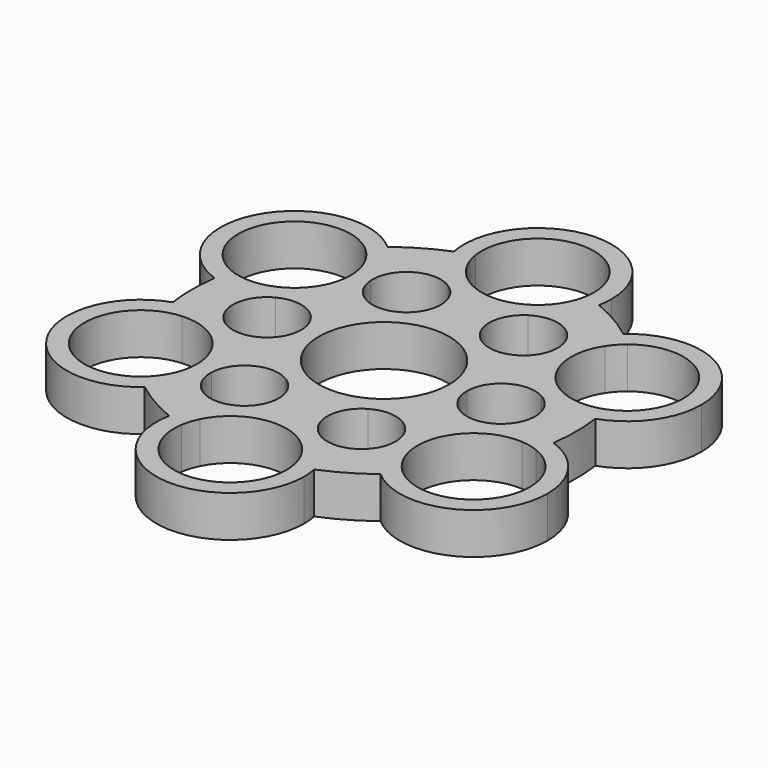
from build123d import *

# Parameters (mm, degrees)
F0_R     = 11
F1_DEPTH = 7


with BuildPart() as f1:
    # F0 (on Top) → F1 (new body)
    with BuildSketch(Plane.XY):
        with BuildLine():
            ThreePointArc((7.0000001006, -12.1243555949), (12.124355682, -6.9999999497), (14, 0))
            ThreePointArc((14, 0), (12.1243557011, 6.9999999166), (7.0000001668, 12.1243555567))
            ThreePointArc((7.0000001668, 12.1243555567), (0.1361246737, 13.9993382013), (-6.7629128968, 12.2581813149))
            ThreePointArc((-6.7629128968, 12.2581813149), (-6.99546954, 12.1165086661), (-7.2344399745, 11.9859450297))
            ThreePointArc((-7.2344399745, 11.9859450297), (-12.191844808, 6.881781759), (-14, 0))
            ThreePointArc((-14, 0), (-12.1243555958, -7.000000099), (-6.999999802, -12.1243557673))
            ThreePointArc((-6.999999802, -12.1243557673), (1.724e-07, -14), (7.0000001006, -12.1243555949))
        make_face()
        Circle(F0_R, mode=Mode.SUBTRACT)
        with BuildLine():
            ThreePointArc((22.4231761247, -5.1368869024), (16.769566617, -4.9329885231), (14, 0))
            ThreePointArc((14, 0), (12.124355682, -6.9999999497), (7.0000001006, -12.1243555949))
            ThreePointArc((7.0000001006, -12.1243555949), (12.6568763598, -12.0563762611), (15.6602625749, -16.8505958477))
            ThreePointArc((15.6602625749, -16.8505958477), (17.3205082906, -9.9999996277), (22.4231761247, -5.1368869024))
        make_face()
        with BuildLine():
            ThreePointArc((7.0000001668, 12.1243555567), (12.1243557011, 6.9999999166), (14, 0))
            ThreePointArc((14, 0), (16.769566627, 4.9329885292), (22.4231761455, 5.1368868917))
            ThreePointArc((22.4231761455, 5.1368868917), (17.3205082443, 9.9999997079), (15.6602625849, 16.8505960559))
            ThreePointArc((15.6602625849, 16.8505960559), (12.6568764848, 12.0563763294), (7.0000001668, 12.1243555567))
        make_face()
        with BuildLine():
            ThreePointArc((-6.7629128968, 12.2581813149), (0.1361246737, 13.9993382013), (7.0000001668, 12.1243555567))
            ThreePointArc((7.0000001668, 12.1243555567), (4.1126899405, 16.9893645646), (6.7629130014, 21.9874832825))
            ThreePointArc((6.7629130014, 21.9874832825), (0.0018890383, 20.0000001427), (-6.759735325, 21.9854396984))
            ThreePointArc((-6.759735325, 21.9854396984), (-4.8119543875, 19.8928592028), (-4.1050678819, 17.1228311923))
            ThreePointArc((-4.1050678819, 17.1228311923), (-4.8128595342, 14.3511458497), (-6.7629128968, 12.2581813149))
        make_face()
        with BuildLine():
            ThreePointArc((6.7629128862, -21.9874832084), (4.1126899412, -16.9893645344), (7.0000001006, -12.1243555949))
            ThreePointArc((7.0000001006, -12.1243555949), (1.724e-07, -14), (-6.999999802, -12.1243557673))
            ThreePointArc((-6.999999802, -12.1243557673), (-4.8851208082, -14.2392348866), (-4.1110213762, -17.1282134114))
            ThreePointArc((-4.1110213762, -17.1282134114), (-4.8171414782, -19.8961111559), (-6.7629128995, -21.987483217))
            ThreePointArc((-6.7629128995, -21.987483217), (-7.9e-09, -20), (6.7629128862, -21.9874832084))
        make_face()
        with BuildLine():
            ThreePointArc((15.6602625849, 16.8505960559), (17.3205082443, 9.9999997079), (22.4231761455, 5.1368868917))
            ThreePointArc((22.4231761455, 5.1368868917), (25.7437624558, 3.9829672479), (29.2543281187, 3.7992481264))
            ThreePointArc((29.2543281187, 3.7992481264), (29.0218126442, 5.2900274902), (28.7133790239, 6.7669686736))
            ThreePointArc((28.7133790239, 6.7669686736), (19.918584287, 11.5), (20.2170562899, 21.4830313264))
            ThreePointArc((20.2170562899, 21.4830313264), (19.0922045153, 22.4886132686), (17.9174094521, 23.4353672582))
            ThreePointArc((17.9174094521, 23.4353672582), (16.3212319377, 20.3032683327), (15.6602625849, 16.8505960559))
        make_face()
        with BuildLine():
            ThreePointArc((29.2543281187, 3.7992481264), (25.7437624558, 3.9829672479), (22.4231761455, 5.1368868917))
            ThreePointArc((22.4231761455, 5.1368868917), (24.7109457768, 3.0083906207), (25.5559144953, 0))
            ThreePointArc((25.5559144953, 0), (24.7109457708, -3.0083906307), (22.4231761247, -5.1368869024))
            ThreePointArc((22.4231761247, -5.1368869024), (25.7437624444, -3.9829672502), (29.2543281187, -3.7992481264))
            ThreePointArc((29.2543281187, -3.7992481264), (29.5, 0), (29.2543281187, 3.7992481264))
        make_face()
        with BuildLine():
            ThreePointArc((29.2543281187, -3.7992481264), (25.7437624444, -3.9829672502), (22.4231761247, -5.1368869024))
            ThreePointArc((22.4231761247, -5.1368869024), (17.3205082906, -9.9999996277), (15.6602625749, -16.8505958477))
            ThreePointArc((15.6602625749, -16.8505958477), (16.3212319039, -20.3032682341), (17.9174094521, -23.4353672582))
            ThreePointArc((17.9174094521, -23.4353672582), (19.0922045153, -22.4886132686), (20.2170562899, -21.4830313264))
            ThreePointArc((20.2170562899, -21.4830313264), (19.918584287, -11.5), (28.7133790239, -6.7669686736))
            ThreePointArc((28.7133790239, -6.7669686736), (29.0218126442, -5.2900274902), (29.2543281187, -3.7992481264))
        make_face()
        with BuildLine():
            ThreePointArc((-6.759735325, 21.9854396984), (0.0018890383, 20.0000001427), (6.7629130014, 21.9874832825))
            ThreePointArc((6.7629130014, 21.9874832825), (9.422530203, 24.2862356636), (11.3369186666, 27.2346153846))
            ThreePointArc((11.3369186666, 27.2346153846), (9.9296081288, 27.7786407588), (8.496322734, 28.25))
            ThreePointArc((8.496322734, 28.25), (0, 23), (-8.496322734, 28.25))
            ThreePointArc((-8.496322734, 28.25), (-9.9296081288, 27.7786407588), (-11.3369186666, 27.2346153846))
            ThreePointArc((-11.3369186666, 27.2346153846), (-9.4212888061, 24.2848117957), (-6.759735325, 21.9854396984))
        make_face()
        with BuildLine():
            ThreePointArc((11.3369186666, 27.2346153846), (9.422530203, 24.2862356636), (6.7629130014, 21.9874832825))
            ThreePointArc((6.7629130014, 21.9874832825), (12.6568764214, 22.2000505281), (15.6669358715, 17.1282134114))
            ThreePointArc((15.6669358715, 17.1282134114), (15.6652673089, 16.9893646368), (15.6602625849, 16.8505960559))
            ThreePointArc((15.6602625849, 16.8505960559), (16.3212319377, 20.3032683327), (17.9174094521, 23.4353672582))
            ThreePointArc((17.9174094521, 23.4353672582), (14.75, 25.5477494116), (11.3369186666, 27.2346153846))
        make_face()
        with BuildLine():
            ThreePointArc((-15.6602625894, -16.850596149), (-12.6568763408, -12.0563762508), (-6.999999802, -12.1243557673))
            ThreePointArc((-6.999999802, -12.1243557673), (-12.1243555958, -7.000000099), (-14, 0))
            ThreePointArc((-14, 0), (-16.7695666992, -4.9329885732), (-22.4231762959, -5.1368868142))
            ThreePointArc((-22.4231762959, -5.1368868143), (-17.4738268273, -9.741663676), (-15.645825623, -16.25))
            ThreePointArc((-15.645825623, -16.25), (-15.6494353858, -16.5503848199), (-15.6602625894, -16.850596149))
        make_face()
        with BuildLine():
            ThreePointArc((17.9174094521, -23.4353672582), (16.3212319039, -20.3032682341), (15.6602625749, -16.8505958477))
            ThreePointArc((15.6602625749, -16.8505958477), (15.6652673064, -16.9893645326), (15.6669358715, -17.1282134114))
            ThreePointArc((15.6669358715, -17.1282134114), (12.6568763613, -22.2000505609), (6.7629128862, -21.9874832084))
            ThreePointArc((6.7629128862, -21.9874832084), (9.422530158, -24.286235612), (11.3369186666, -27.2346153846))
            ThreePointArc((11.3369186666, -27.2346153846), (14.75, -25.5477494116), (17.9174094521, -23.4353672582))
        make_face()
        with BuildLine():
            ThreePointArc((11.3369186666, -27.2346153846), (9.422530158, -24.286235612), (6.7629128862, -21.9874832084))
            ThreePointArc((6.7629128862, -21.9874832084), (-7.9e-09, -20), (-6.7629128995, -21.987483217))
            ThreePointArc((-6.7629128995, -21.987483217), (-9.4225301632, -24.286235618), (-11.3369186666, -27.2346153846))
            ThreePointArc((-11.3369186666, -27.2346153846), (-9.9296081288, -27.7786407588), (-8.496322734, -28.25))
            ThreePointArc((-8.496322734, -28.25), (0, -23), (8.496322734, -28.25))
            ThreePointArc((8.496322734, -28.25), (9.9296081288, -27.7786407588), (11.3369186666, -27.2346153846))
        make_face()
        with BuildLine():
            ThreePointArc((28.7133790239, 6.7669686736), (29.0218126442, 5.2900274902), (29.2543281187, 3.7992481264))
            ThreePointArc((29.2543281187, 3.7992481264), (30.7447425948, 4.0231594198), (32.1973755284, 4.4248174067))
            ThreePointArc((32.1973755284, 4.4248174067), (31.9549148923, 5.9273446187), (31.642376555, 7.4168730576))
            ThreePointArc((31.642376555, 7.4168730576), (30.2036958653, 6.9755636254), (28.7133790239, 6.7669686736))
        make_face()
        with BuildLine():
            ThreePointArc((32.1973755284, 4.4248174067), (30.7447425948, 4.0231594198), (29.2543281187, 3.7992481264))
            ThreePointArc((29.2543281187, 3.7992481264), (29.5, 0), (29.2543281187, -3.7992481264))
            ThreePointArc((29.2543281187, -3.7992481264), (30.7447425948, -4.0231594198), (32.1973755284, -4.4248174067))
            ThreePointArc((32.1973755284, -4.4248174067), (32.5, 0), (32.1973755284, 4.4248174067))
        make_face()
        with BuildLine():
            ThreePointArc((32.1973755284, -4.4248174067), (30.7447425948, -4.0231594198), (29.2543281187, -3.7992481264))
            ThreePointArc((29.2543281187, -3.7992481264), (29.0218126442, -5.2900274902), (28.7133790239, -6.7669686736))
            ThreePointArc((28.7133790239, -6.7669686736), (30.2036958653, -6.9755636254), (31.642376555, -7.4168730576))
            ThreePointArc((31.642376555, -7.4168730576), (31.9549148923, -5.9273446187), (32.1973755284, -4.4248174067))
        make_face()
        with BuildLine():
            ThreePointArc((-14, 0), (-12.191844808, 6.881781759), (-7.2344399745, 11.9859450297))
            ThreePointArc((-7.2344399745, 11.9859450297), (-12.7746372788, 12.1155647212), (-15.660081627, 16.8468223075))
            ThreePointArc((-15.660081627, 16.8468223075), (-15.6493901322, 16.5484962731), (-15.645825623, 16.25))
            ThreePointArc((-15.645825623, 16.25), (-17.473826823, 9.7416636832), (-22.423176281, 5.1368868219))
            ThreePointArc((-22.423176281, 5.1368868219), (-16.769566692, 4.9329885689), (-14, 0))
        make_face()
        with BuildLine():
            ThreePointArc((-15.660081627, 16.8468223075), (-12.7762728806, 22.1291537044), (-6.759735325, 21.9854396984))
            ThreePointArc((-6.759735325, 21.9854396984), (-9.4212888061, 24.2848117957), (-11.3369186666, 27.2346153846))
            ThreePointArc((-11.3369186666, 27.2346153846), (-14.75, 25.5477494116), (-17.9174094521, 23.4353672582))
            ThreePointArc((-17.9174094521, 23.4353672582), (-16.3206195291, 20.3014813138), (-15.660081627, 16.8468223075))
        make_face()
        with BuildLine():
            ThreePointArc((8.496322734, 28.25), (9.9296081288, 27.7786407588), (11.3369186666, 27.2346153846))
            ThreePointArc((11.3369186666, 27.2346153846), (11.8882130364, 28.6373078299), (12.2666834829, 30.0961538462))
            ThreePointArc((12.2666834829, 30.0961538462), (10.8442264294, 30.6374403818), (9.3979877929, 31.1115384615))
            ThreePointArc((9.3979877929, 31.1115384615), (9.0608326273, 29.6449497203), (8.496322734, 28.25))
        make_face()
        with BuildLine():
            ThreePointArc((12.2666834829, 30.0961538462), (11.8882130364, 28.6373078299), (11.3369186666, 27.2346153846))
            ThreePointArc((11.3369186666, 27.2346153846), (14.75, 25.5477494116), (17.9174094521, 23.4353672582))
            ThreePointArc((17.9174094521, 23.4353672582), (18.8565295584, 24.61414841), (19.9306920455, 25.6713364394))
            ThreePointArc((19.9306920455, 25.6713364394), (16.25, 28.145825623), (12.2666834829, 30.0961538462))
        make_face()
        with BuildLine():
            ThreePointArc((19.9306920455, 25.6713364394), (18.8565295584, 24.61414841), (17.9174094521, 23.4353672582))
            ThreePointArc((17.9174094521, 23.4353672582), (19.0922045153, 22.4886132686), (20.2170562899, 21.4830313264))
            ThreePointArc((20.2170562899, 21.4830313264), (21.142863238, 22.6693860948), (22.244388762, 23.6946654039))
            ThreePointArc((22.244388762, 23.6946654039), (21.1106884629, 24.7100957631), (19.9306920455, 25.6713364394))
        make_face()
        with BuildLine():
            ThreePointArc((-6.7629128995, -21.987483217), (-12.7779571757, -22.1320712114), (-15.6602625894, -16.850596149))
            ThreePointArc((-15.6602625894, -16.850596149), (-16.3212319528, -20.3032683768), (-17.9174094521, -23.4353672582))
            ThreePointArc((-17.9174094521, -23.4353672582), (-14.75, -25.5477494116), (-11.3369186666, -27.2346153846))
            ThreePointArc((-11.3369186666, -27.2346153846), (-9.4225301632, -24.286235618), (-6.7629128995, -21.987483217))
        make_face()
        with BuildLine():
            ThreePointArc((-17.9174094521, -23.4353672582), (-16.3212319528, -20.3032683768), (-15.6602625894, -16.850596149))
            ThreePointArc((-15.6602625894, -16.850596149), (-15.6494353858, -16.5503848199), (-15.645825623, -16.25))
            ThreePointArc((-15.645825623, -16.25), (-17.4738268273, -9.741663676), (-22.4231762959, -5.1368868143))
            ThreePointArc((-22.4231762959, -5.1368868143), (-25.7437625388, -3.9829672317), (-29.2543281187, -3.7992481264))
            ThreePointArc((-29.2543281187, -3.7992481264), (-29.0218126442, -5.2900274902), (-28.7133790239, -6.7669686736))
            ThreePointArc((-28.7133790239, -6.7669686736), (-21.6320616308, -9.3347358218), (-18.645825623, -16.25))
            ThreePointArc((-18.645825623, -16.25), (-19.0471084424, -18.9819124561), (-20.2170562899, -21.4830313264))
            ThreePointArc((-20.2170562899, -21.4830313264), (-19.0922045153, -22.4886132686), (-17.9174094521, -23.4353672582))
        make_face()
        with BuildLine():
            ThreePointArc((20.2170562899, -21.4830313264), (19.0922045153, -22.4886132686), (17.9174094521, -23.4353672582))
            ThreePointArc((17.9174094521, -23.4353672582), (18.8565295584, -24.61414841), (19.9306920455, -25.6713364394))
            ThreePointArc((19.9306920455, -25.6713364394), (21.1106884629, -24.7100957631), (22.244388762, -23.6946654039))
            ThreePointArc((22.244388762, -23.6946654039), (21.142863238, -22.6693860948), (20.2170562899, -21.4830313264))
        make_face()
        with BuildLine():
            ThreePointArc((19.9306920455, -25.6713364394), (18.8565295584, -24.61414841), (17.9174094521, -23.4353672582))
            ThreePointArc((17.9174094521, -23.4353672582), (14.75, -25.5477494116), (11.3369186666, -27.2346153846))
            ThreePointArc((11.3369186666, -27.2346153846), (11.8882130364, -28.6373078299), (12.2666834829, -30.0961538462))
            ThreePointArc((12.2666834829, -30.0961538462), (16.25, -28.145825623), (19.9306920455, -25.6713364394))
        make_face()
        with BuildLine():
            ThreePointArc((12.2666834829, -30.0961538462), (11.8882130364, -28.6373078299), (11.3369186666, -27.2346153846))
            ThreePointArc((11.3369186666, -27.2346153846), (9.9296081288, -27.7786407588), (8.496322734, -28.25))
            ThreePointArc((8.496322734, -28.25), (9.0608326273, -29.6449497203), (9.3979877929, -31.1115384615))
            ThreePointArc((9.3979877929, -31.1115384615), (10.8442264294, -30.6374403818), (12.2666834829, -30.0961538462))
        make_face()
        with BuildLine():
            ThreePointArc((31.642376555, 7.4168730576), (31.9549148923, 5.9273446187), (32.1973755284, 4.4248174067))
            ThreePointArc((32.1973755284, 4.4248174067), (38.3167246447, 8.9834455833), (40.645825623, 16.25))
            ThreePointArc((40.645825623, 16.25), (33.3208053467, 27.6284702337), (19.9306920455, 25.6713364394))
            ThreePointArc((19.9306920455, 25.6713364394), (21.1106884629, 24.7100957631), (22.244388762, 23.6946654039))
            ThreePointArc((22.244388762, 23.6946654039), (32.2802149262, 24.8031763158), (37.645825623, 16.25))
            ThreePointArc((37.645825623, 16.25), (36.0028999466, 10.9099266791), (31.642376555, 7.4168730576))
        make_face()
        with BuildLine():
            ThreePointArc((40.645825623, -16.25), (38.3167246447, -8.9834455833), (32.1973755284, -4.4248174067))
            ThreePointArc((32.1973755284, -4.4248174067), (31.9549148923, -5.9273446187), (31.642376555, -7.4168730576))
            ThreePointArc((31.642376555, -7.4168730576), (36.0028999466, -10.9099266791), (37.645825623, -16.25))
            ThreePointArc((37.645825623, -16.25), (32.2802149262, -24.8031763158), (22.244388762, -23.6946654039))
            ThreePointArc((22.244388762, -23.6946654039), (21.1106884629, -24.7100957631), (19.9306920455, -25.6713364394))
            ThreePointArc((19.9306920455, -25.6713364394), (33.3208053467, -27.6284702337), (40.645825623, -16.25))
        make_face()
        with BuildLine():
            ThreePointArc((-15.645825623, 16.25), (-15.6493901322, 16.5484962731), (-15.660081627, 16.8468223075))
            ThreePointArc((-15.660081627, 16.8468223075), (-16.3206195291, 20.3014813138), (-17.9174094521, 23.4353672582))
            ThreePointArc((-17.9174094521, 23.4353672582), (-19.0922045153, 22.4886132686), (-20.2170562899, 21.4830313264))
            ThreePointArc((-20.2170562899, 21.4830313264), (-19.0471084424, 18.9819124561), (-18.645825623, 16.25))
            ThreePointArc((-18.645825623, 16.25), (-21.6320616308, 9.3347358218), (-28.7133790239, 6.7669686736))
            ThreePointArc((-28.7133790239, 6.7669686736), (-29.0218126442, 5.2900274902), (-29.2543281187, 3.7992481264))
            ThreePointArc((-29.2543281187, 3.7992481264), (-25.7437625306, 3.9829672333), (-22.423176281, 5.1368868219))
            ThreePointArc((-22.423176281, 5.1368868219), (-17.473826823, 9.7416636832), (-15.645825623, 16.25))
        make_face()
        with BuildLine():
            ThreePointArc((-17.9174094521, 23.4353672582), (-14.75, 25.5477494116), (-11.3369186666, 27.2346153846))
            ThreePointArc((-11.3369186666, 27.2346153846), (-11.8882130364, 28.6373078299), (-12.2666834829, 30.0961538462))
            ThreePointArc((-12.2666834829, 30.0961538462), (-16.25, 28.145825623), (-19.9306920455, 25.6713364394))
            ThreePointArc((-19.9306920455, 25.6713364394), (-18.8565295584, 24.61414841), (-17.9174094521, 23.4353672582))
        make_face()
        with BuildLine():
            ThreePointArc((-12.2666834829, 30.0961538462), (-11.8882130364, 28.6373078299), (-11.3369186666, 27.2346153846))
            ThreePointArc((-11.3369186666, 27.2346153846), (-9.9296081288, 27.7786407588), (-8.496322734, 28.25))
            ThreePointArc((-8.496322734, 28.25), (-9.0608326273, 29.6449497203), (-9.3979877929, 31.1115384615))
            ThreePointArc((-9.3979877929, 31.1115384615), (-10.8442264294, 30.6374403818), (-12.2666834829, 30.0961538462))
        make_face()
        with BuildLine():
            ThreePointArc((9.3979877929, 31.1115384615), (10.8442264294, 30.6374403818), (12.2666834829, 30.0961538462))
            ThreePointArc((12.2666834829, 30.0961538462), (12.4415341404, 31.292428788), (12.5, 32.5))
            ThreePointArc((12.5, 32.5), (-1.207571212, 44.9415341404), (-12.2666834829, 30.0961538462))
            ThreePointArc((-12.2666834829, 30.0961538462), (-10.8442264294, 30.6374403818), (-9.3979877929, 31.1115384615))
            ThreePointArc((-9.3979877929, 31.1115384615), (-0.6961019922, 41.9744626242), (9.5, 32.5))
            ThreePointArc((9.5, 32.5), (9.4744626242, 31.8038980078), (9.3979877929, 31.1115384615))
        make_face()
        with BuildLine():
            ThreePointArc((-22.4231762959, -5.1368868142), (-25.5559144953, 8.4e-09), (-22.423176281, 5.1368868219))
            ThreePointArc((-22.423176281, 5.1368868219), (-25.7437625306, 3.9829672333), (-29.2543281187, 3.7992481264))
            ThreePointArc((-29.2543281187, 3.7992481264), (-29.5, 0), (-29.2543281187, -3.7992481264))
            ThreePointArc((-29.2543281187, -3.7992481264), (-25.7437625388, -3.9829672317), (-22.4231762959, -5.1368868143))
        make_face()
        with BuildLine():
            ThreePointArc((-11.3369186666, -27.2346153846), (-14.75, -25.5477494116), (-17.9174094521, -23.4353672582))
            ThreePointArc((-17.9174094521, -23.4353672582), (-18.8565295584, -24.61414841), (-19.9306920455, -25.6713364394))
            ThreePointArc((-19.9306920455, -25.6713364394), (-16.25, -28.145825623), (-12.2666834829, -30.0961538462))
            ThreePointArc((-12.2666834829, -30.0961538462), (-11.8882130364, -28.6373078299), (-11.3369186666, -27.2346153846))
        make_face()
        with BuildLine():
            ThreePointArc((-19.9306920455, -25.6713364394), (-18.8565295584, -24.61414841), (-17.9174094521, -23.4353672582))
            ThreePointArc((-17.9174094521, -23.4353672582), (-19.0922045153, -22.4886132686), (-20.2170562899, -21.4830313264))
            ThreePointArc((-20.2170562899, -21.4830313264), (-21.142863238, -22.6693860948), (-22.244388762, -23.6946654039))
            ThreePointArc((-22.244388762, -23.6946654039), (-21.1106884629, -24.7100957631), (-19.9306920455, -25.6713364394))
        make_face()
        with BuildLine():
            ThreePointArc((12.5, -32.5), (12.4415341404, -31.292428788), (12.2666834829, -30.0961538462))
            ThreePointArc((12.2666834829, -30.0961538462), (10.8442264294, -30.6374403818), (9.3979877929, -31.1115384615))
            ThreePointArc((9.3979877929, -31.1115384615), (9.4744626242, -31.8038980078), (9.5, -32.5))
            ThreePointArc((9.5, -32.5), (-0.6961019922, -41.9744626242), (-9.3979877929, -31.1115384615))
            ThreePointArc((-9.3979877929, -31.1115384615), (-10.8442264294, -30.6374403818), (-12.2666834829, -30.0961538462))
            ThreePointArc((-12.2666834829, -30.0961538462), (-1.207571212, -44.9415341404), (12.5, -32.5))
        make_face()
        with BuildLine():
            ThreePointArc((-8.496322734, -28.25), (-9.9296081288, -27.7786407588), (-11.3369186666, -27.2346153846))
            ThreePointArc((-11.3369186666, -27.2346153846), (-11.8882130364, -28.6373078299), (-12.2666834829, -30.0961538462))
            ThreePointArc((-12.2666834829, -30.0961538462), (-10.8442264294, -30.6374403818), (-9.3979877929, -31.1115384615))
            ThreePointArc((-9.3979877929, -31.1115384615), (-9.0608326273, -29.6449497203), (-8.496322734, -28.25))
        make_face()
        with BuildLine():
            ThreePointArc((-20.2170562899, 21.4830313264), (-19.0922045153, 22.4886132686), (-17.9174094521, 23.4353672582))
            ThreePointArc((-17.9174094521, 23.4353672582), (-18.8565295584, 24.61414841), (-19.9306920455, 25.6713364394))
            ThreePointArc((-19.9306920455, 25.6713364394), (-21.1106884629, 24.7100957631), (-22.244388762, 23.6946654039))
            ThreePointArc((-22.244388762, 23.6946654039), (-21.142863238, 22.6693860948), (-20.2170562899, 21.4830313264))
        make_face()
        with BuildLine():
            ThreePointArc((-32.1973755284, 4.4248174067), (-30.7447425948, 4.0231594198), (-29.2543281187, 3.7992481264))
            ThreePointArc((-29.2543281187, 3.7992481264), (-29.0218126442, 5.2900274902), (-28.7133790239, 6.7669686736))
            ThreePointArc((-28.7133790239, 6.7669686736), (-30.2036958653, 6.9755636254), (-31.642376555, 7.4168730576))
            ThreePointArc((-31.642376555, 7.4168730576), (-31.9549148923, 5.9273446187), (-32.1973755284, 4.4248174067))
        make_face()
        with BuildLine():
            ThreePointArc((-29.2543281187, -3.7992481264), (-29.5, 0), (-29.2543281187, 3.7992481264))
            ThreePointArc((-29.2543281187, 3.7992481264), (-30.7447425948, 4.0231594198), (-32.1973755284, 4.4248174067))
            ThreePointArc((-32.1973755284, 4.4248174067), (-32.5, 0), (-32.1973755284, -4.4248174067))
            ThreePointArc((-32.1973755284, -4.4248174067), (-30.7447425948, -4.0231594198), (-29.2543281187, -3.7992481264))
        make_face()
        with BuildLine():
            ThreePointArc((-28.7133790239, -6.7669686736), (-29.0218126442, -5.2900274902), (-29.2543281187, -3.7992481264))
            ThreePointArc((-29.2543281187, -3.7992481264), (-30.7447425948, -4.0231594198), (-32.1973755284, -4.4248174067))
            ThreePointArc((-32.1973755284, -4.4248174067), (-31.9549148923, -5.9273446187), (-31.642376555, -7.4168730576))
            ThreePointArc((-31.642376555, -7.4168730576), (-30.2036958653, -6.9755636254), (-28.7133790239, -6.7669686736))
        make_face()
        with BuildLine():
            ThreePointArc((-32.1973755284, -4.4248174067), (-38.9711431703, -22.5), (-19.9306920455, -25.6713364394))
            ThreePointArc((-19.9306920455, -25.6713364394), (-21.1106884629, -24.7100957631), (-22.244388762, -23.6946654039))
            ThreePointArc((-22.244388762, -23.6946654039), (-36.3730669589, -21), (-31.642376555, -7.4168730576))
            ThreePointArc((-31.642376555, -7.4168730576), (-31.9549148923, -5.9273446187), (-32.1973755284, -4.4248174067))
        make_face()
        with BuildLine():
            ThreePointArc((-22.244388762, 23.6946654039), (-21.1106884629, 24.7100957631), (-19.9306920455, 25.6713364394))
            ThreePointArc((-19.9306920455, 25.6713364394), (-38.9711431703, 22.5), (-32.1973755284, 4.4248174067))
            ThreePointArc((-32.1973755284, 4.4248174067), (-31.9549148923, 5.9273446187), (-31.642376555, 7.4168730576))
            ThreePointArc((-31.642376555, 7.4168730576), (-36.3730669589, 21), (-22.244388762, 23.6946654039))
        make_face()
    extrude(amount=F1_DEPTH)


solid = f1.part
